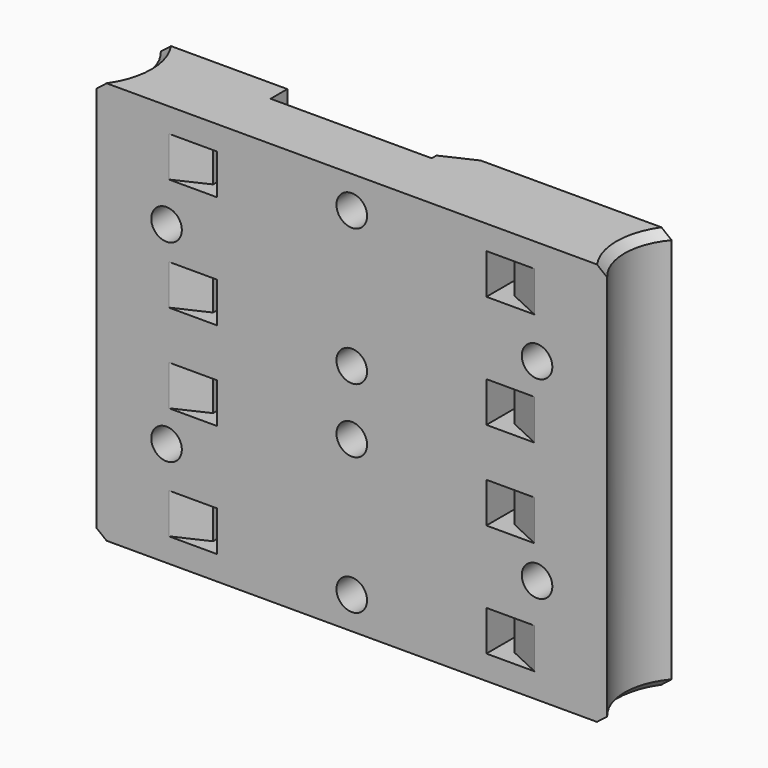
from build123d import *

# Parameters (mm, degrees)
F1_DEPTH     = 12.5
F2_R         = 1.9
F2_W         = 2
F2_H         = 5
F3_DEPTH     = 25
F5_T1_DEPTH  = 5
F5_T3_DEPTH  = 5
F5_T5_DEPTH  = 22.8639018857
F5_T7_DEPTH  = 22.8639018857
F5_T12_DEPTH = 25.7278037714
F5_T17_DEPTH = 25.7278037714
F5_T22_DEPTH = 25.7278037714
F5_T27_DEPTH = 25.7278037714
F5_T32_DEPTH = 25.7278037714
F5_T37_DEPTH = 25.7278037714
F5_T42_DEPTH = 25.7278037714
F5_T47_DEPTH = 25.7278037714
F10_SIZE     = 1


# Not quite as in the source:
# - a fillet or chamfer that OpenCascade refuses, or shapes differently, is made with other operations: its cross-section is extruded or revolved along the edge and cut away or added
# - two fillets or chamfers of one size are made in one step


with BuildPart() as f1:
    # F0 (on Top) → F1 (new body, symmetric)
    with BuildSketch(Plane.XY):
        with BuildLine():
            ThreePointArc((-31.711398723, 5), (-30.3486184122, 2.6632855775), (-29.875, 0))
            ThreePointArc((-29.875, 0), (-30.3486184122, -2.6632855775), (-31.711398723, -5))
            Line((-31.711398723, -5), (31.711398723, -5))
            ThreePointArc((31.711398723, -5), (29.875, 0), (31.711398723, 5))
            Line((31.711398723, 5), (4, 5))
            Line((4, 5), (4, 2.4))
            Line((4, 2.4), (-16, 2.4))
            Line((-16, 2.4), (-16, 5))
            Line((-16, 5), (-31.711398723, 5))
        make_face()
    extrude(amount=F1_DEPTH, both=True)

    # F2 (on face) → F3 (cut)
    with BuildSketch(Plane.XZ.offset(5)):
        with Locations((0, 8.5)):
            Circle(F2_R)
        with Locations((0, -8.5)):
            Circle(F2_R)
        with Locations((-17.711398723, 7)):
            Rectangle(F2_W, F2_H)
        with Locations((-17.711398723, -7)):
            Rectangle(F2_W, F2_H)
        with Locations((17.711398723, 7)):
            Rectangle(F2_W, F2_H)
        with Locations((17.711398723, -7)):
            Rectangle(F2_W, F2_H)
        with Locations((-23, 0.5)):
            Circle(F2_R)
        with Locations((23, 0.5)):
            Circle(F2_R)
    extrude(amount=-F3_DEPTH, mode=Mode.SUBTRACT)

    # F5: chamfer of 4 x 1.8652306326 on 10 edges, made by hand

    # F5_s2 → F5_t1 (cut)
    with BuildSketch(Plane.XY.offset(-9.5)):
        Polygon((22.711398723, -5), (18.711398723, -3.1347693674), (18.711398723, -5), align=None)
        Polygon((-22.711398723, -5), (-18.711398723, -3.1347693674), (-18.711398723, -5), align=None)
        Polygon((-18.711398723, 3.1347693674), (-22.711398723, 5), (-18.711398723, 5), align=None)
        Polygon((18.711398723, 3.1347693674), (22.711398723, 5), (18.711398723, 5), align=None)
    extrude(amount=F5_T1_DEPTH, mode=Mode.SUBTRACT)

    # F5_s4 → F5_t3 (cut)
    with BuildSketch(Plane.XY.offset(4.5)):
        Polygon((22.711398723, -5), (18.711398723, -3.1347693674), (18.711398723, -5), align=None)
        Polygon((-22.711398723, -5), (-18.711398723, -3.1347693674), (-18.711398723, -5), align=None)
        Polygon((-18.711398723, 3.1347693674), (-22.711398723, 5), (-18.711398723, 5), align=None)
        Polygon((18.711398723, 3.1347693674), (22.711398723, 5), (18.711398723, 5), align=None)
    extrude(amount=F5_T3_DEPTH, mode=Mode.SUBTRACT)

    # F5_s6 → F5_t5 (cut)
    with BuildSketch(Plane.XY.offset(-22.8639018857)):
        Polygon((8, 5), (4, 3.1347693674), (4, 5), align=None)
    extrude(amount=F5_T5_DEPTH, mode=Mode.SUBTRACT)

    # F5_s8 → F5_t7 (cut)
    with BuildSketch(Plane.XY):
        Polygon((8, 5), (4, 3.1347693674), (4, 5), align=None)
    extrude(amount=F5_T7_DEPTH, mode=Mode.SUBTRACT)


with BuildPart() as f5_tool10:
    # F5_s11 → F5_t12 (new body)
    with BuildSketch(Plane.XY.offset(-19.8639018857)):
        Polygon((22.711398723, -5), (18.711398723, -3.1347693674), (18.711398723, -5), align=None)
    extrude(amount=F5_T12_DEPTH)

    split(bisect_by=Plane.XY.offset(4.5), keep=Keep.TOP)


with BuildPart() as f1_1:
    add(f1.part)

    # F5_t9: cut F5_tool10
    add(f5_tool10.part, mode=Mode.SUBTRACT)


with BuildPart() as f5_tool15:
    # F5_s16 → F5_t17 (new body)
    with BuildSketch(Plane.XY.offset(-5.8639018857)):
        Polygon((22.711398723, -5), (18.711398723, -3.1347693674), (18.711398723, -5), align=None)
    extrude(amount=F5_T17_DEPTH)

    split(bisect_by=Plane.XY.offset(-4.5), keep=Keep.BOTTOM)


with BuildPart() as f1_2:
    add(f1_1.part)

    # F5_t14: cut F5_tool15
    add(f5_tool15.part, mode=Mode.SUBTRACT)


with BuildPart() as f5_tool20:
    # F5_s21 → F5_t22 (new body)
    with BuildSketch(Plane.XY.offset(5.8639018857)):
        Polygon((-22.711398723, -5), (-18.711398723, -3.1347693674), (-18.711398723, -5), align=None)
    extrude(amount=-F5_T22_DEPTH)

    split(bisect_by=Plane.XY.offset(4.5), keep=Keep.TOP)


with BuildPart() as f1_3:
    add(f1_2.part)

    # F5_t19: cut F5_tool20
    add(f5_tool20.part, mode=Mode.SUBTRACT)


with BuildPart() as f5_tool25:
    # F5_s26 → F5_t27 (new body)
    with BuildSketch(Plane.XY.offset(19.8639018857)):
        Polygon((-22.711398723, -5), (-18.711398723, -3.1347693674), (-18.711398723, -5), align=None)
    extrude(amount=-F5_T27_DEPTH)

    split(bisect_by=Plane.XY.offset(-4.5), keep=Keep.BOTTOM)


with BuildPart() as f1_4:
    add(f1_3.part)

    # F5_t24: cut F5_tool25
    add(f5_tool25.part, mode=Mode.SUBTRACT)


with BuildPart() as f5_tool30:
    # F5_s31 → F5_t32 (new body)
    with BuildSketch(Plane.XY.offset(-19.8639018857)):
        Polygon((-18.711398723, 3.1347693674), (-22.711398723, 5), (-18.711398723, 5), align=None)
    extrude(amount=F5_T32_DEPTH)

    split(bisect_by=Plane.XY.offset(4.5), keep=Keep.TOP)


with BuildPart() as f1_5:
    add(f1_4.part)

    # F5_t29: cut F5_tool30
    add(f5_tool30.part, mode=Mode.SUBTRACT)


with BuildPart() as f5_tool35:
    # F5_s36 → F5_t37 (new body)
    with BuildSketch(Plane.XY.offset(5.8639018857)):
        Polygon((18.711398723, 3.1347693674), (22.711398723, 5), (18.711398723, 5), align=None)
    extrude(amount=-F5_T37_DEPTH)

    split(bisect_by=Plane.XY.offset(4.5), keep=Keep.TOP)


with BuildPart() as f1_6:
    add(f1_5.part)

    # F5_t34: cut F5_tool35
    add(f5_tool35.part, mode=Mode.SUBTRACT)


with BuildPart() as f5_tool40:
    # F5_s41 → F5_t42 (new body)
    with BuildSketch(Plane.XY.offset(19.8639018857)):
        Polygon((-18.711398723, 3.1347693674), (-22.711398723, 5), (-18.711398723, 5), align=None)
    extrude(amount=-F5_T42_DEPTH)

    split(bisect_by=Plane.XY.offset(-4.5), keep=Keep.BOTTOM)


with BuildPart() as f1_7:
    add(f1_6.part)

    # F5_t39: cut F5_tool40
    add(f5_tool40.part, mode=Mode.SUBTRACT)


with BuildPart() as f5_tool45:
    # F5_s46 → F5_t47 (new body)
    with BuildSketch(Plane.XY.offset(-5.8639018857)):
        Polygon((18.711398723, 3.1347693674), (22.711398723, 5), (18.711398723, 5), align=None)
    extrude(amount=F5_T47_DEPTH)

    split(bisect_by=Plane.XY.offset(-4.5), keep=Keep.BOTTOM)


with BuildPart() as f1_8:
    add(f1_7.part)

    # F5_t44: cut F5_tool45
    add(f5_tool45.part, mode=Mode.SUBTRACT)

    # F9: F1 across face


with BuildPart() as f1_9:
    add(f1_8.part)
    add(f1_8.part.mirror(Plane(origin=(0.5278701032, -0.3772073921, 12.5), x_dir=(1, 0, 0), z_dir=(0, 0, 1))))

    # F10
    f10_edges = [f1_9.edges().sort_by_distance(p)[0] for p in [
        (29.875, 0, 37.5),
        (29.875, 0, -12.5),
        (-30.348618, 2.663286, 37.5),
        (-30.348618, -2.663286, 37.5),
        (-30.348618, -2.663286, -12.5),
        (-30.348618, 2.663286, -12.5),
    ]]
    chamfer(f10_edges, length=F10_SIZE)


solid = f1_9.part
